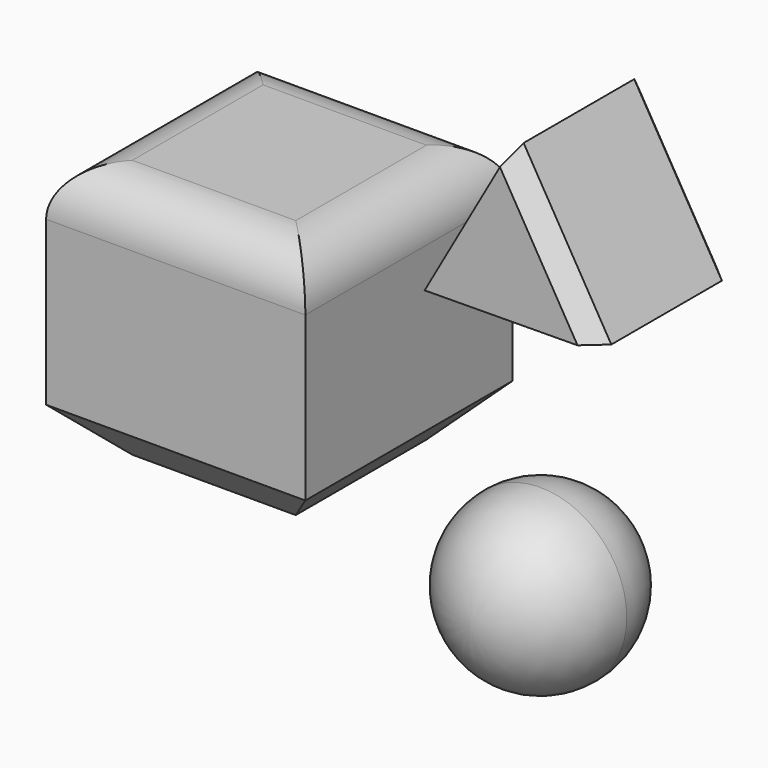
from build123d import *

# Parameters (mm, degrees)
F0_W     = 76.2
F0_H     = 76.2
F1_DEPTH = 76.2
F2_R     = 14.097
F3_SIZE  = 14.097
F4_R     = 25.4
F5_DEPTH = 50.8
F6_R     = 25.39999
F8_DEPTH = 50.8
F9_SIZE2 = 5.08
F9_SIZE  = 5.08


# Not quite as in the source:
# - a fillet or chamfer is up to 0.001 mm smaller than in the source, because OpenCascade refuses the exact size


with BuildPart() as f1:
    # F0 (on Front) → F1 (new body)
    with BuildSketch(Plane.XZ):
        with Locations((-27.5710467249, 19.3739583973)):
            Rectangle(F0_W, F0_H)
    extrude(amount=F1_DEPTH)

    # F2
    f2_edges = [f1.edges().sort_by_distance(p)[0] for p in [
        (-65.671047, -38.1, 57.473958),
        (-27.571047, 0, 57.473958),
        (10.528953, -38.1, 57.473958),
        (-27.571047, -76.2, 57.473958),
    ]]
    fillet(f2_edges, radius=F2_R)

    # F3
    f3_edges = [f1.edges().sort_by_distance(p)[0] for p in [
        (-65.671047, -38.1, -18.726042),
        (-27.571047, -76.2, -18.726042),
        (10.528953, -38.1, -18.726042),
        (-27.571047, 0, -18.726042),
    ]]
    chamfer(f3_edges, length=F3_SIZE)


with BuildPart() as f5:
    # F4 (on Front) → F5 (new body)
    with BuildSketch(Plane.XZ):
        with Locations((38.9659069479, -38.0307249725)):
            Circle(F4_R)
    extrude(amount=F5_DEPTH)

    # F6 (radius 25.4 in the source; OpenCascade refuses exactly that, so slightly less here)
    f6_edges = [f5.edges().sort_by_distance(p)[0] for p in [
        (13.565907, -50.8, -38.030725),
        (13.565907, 0, -38.030725),
    ]]
    fillet(f6_edges, radius=F6_R)


with BuildPart() as f8:
    # F7 (on Front) → F8 (new body)
    with BuildSketch(Plane.XZ):
        Polygon((76.0843477927, 44.654974036), (50.3064604832, 88.4287164607), (25.2862311795, 44.2175399825), align=None)
    extrude(amount=F8_DEPTH)

    # F9
    f9_edges = [f8.edges().sort_by_distance(p)[0] for p in [
        (63.195404, 0, 66.541845),
        (63.195404, -50.8, 66.541845),
    ]]
    chamfer(f9_edges, length=F9_SIZE, length2=F9_SIZE2)


solid = Compound([f1.part, f5.part, f8.part])
